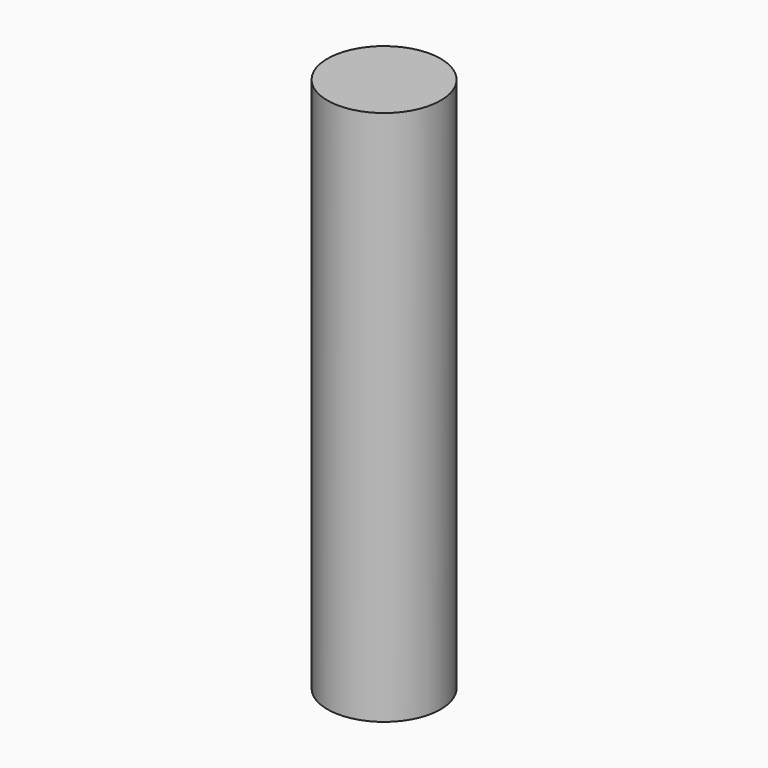
from build123d import *

# Parameters (mm, degrees)
F0_W = 12.7
F0_H = 120.1615070921


# Not quite as in the source:
# - the program builds the solid bodies; features that only make, move or delete a surface that nothing else refers to are left out


with BuildPart() as f1:
    # F0 (on Front) → F1 (revolve)
    with BuildSketch(Plane.XZ):
        Rectangle(F0_W, F0_H)
    revolve(axis=Axis((-6.35, 0, 0), (0, 0, 1)))


solid = f1.part
